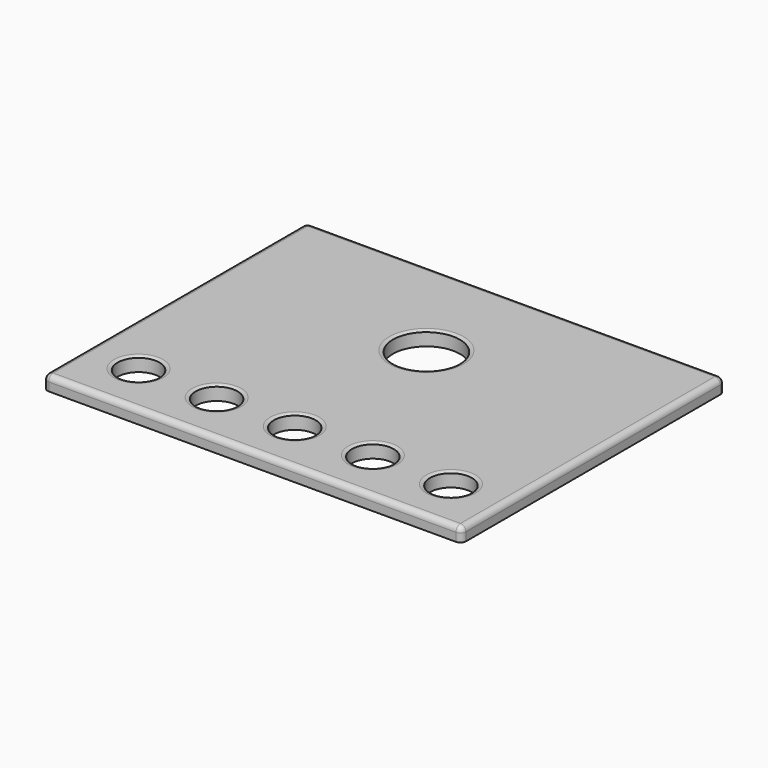
from build123d import *

# Parameters (mm, degrees)
F0_W         = 150
F0_H         = 118
F0_W_2       = 5
F0_H_2       = 5
F0_R         = 7.5
F0_R_2       = 12
F1_DEPTH     = 5
F2_DEPTH     = 1
F3_SIZE      = 0.5
F4_T1_DEPTH  = 160
F4_T3_DEPTH  = 128
F5_T1_DEPTH  = 8
F5_S5_W      = 2
F5_S5_H      = 2
F5_T6_DEPTH  = 2
F5_S11_W     = 2
F5_S11_H     = 2
F5_T12_DEPTH = 2
F5_S17_W     = 2
F5_S17_H     = 2
F5_T18_DEPTH = 2
F5_S23_W     = 2
F5_S23_H     = 2
F5_T24_DEPTH = 2


# Not quite as in the source:
# - a fillet or chamfer that OpenCascade refuses, or shapes differently, is made with other operations: its cross-section is extruded or revolved along the edge and cut away or added


with BuildPart() as f1:
    # F0 (on Top) → F1 (new body)
    with BuildSketch(Plane.XY):
        with Locations((0.2827864019, -6.098040469)):
            Rectangle(F0_W, F0_H)
        with Locations((-67.2172135981, -57.598040469)):
            Rectangle(F0_W_2, F0_H_2, mode=Mode.SUBTRACT)
        with Locations((-55.7172135981, -46.098040469)):
            Circle(F0_R, mode=Mode.SUBTRACT)
        with Locations((-27.7172135981, -46.098040469)):
            Circle(F0_R, mode=Mode.SUBTRACT)
        with Locations((0.2827864019, -46.098040469)):
            Circle(F0_R, mode=Mode.SUBTRACT)
        with Locations((28.2827864019, -46.098040469)):
            Circle(F0_R, mode=Mode.SUBTRACT)
        with Locations((67.7827864019, -57.598040469)):
            Rectangle(F0_W_2, F0_H_2, mode=Mode.SUBTRACT)
        with Locations((56.2827864019, -46.098040469)):
            Circle(F0_R, mode=Mode.SUBTRACT)
        with Locations((-67.2172135981, 45.401959531)):
            Rectangle(F0_W_2, F0_H_2, mode=Mode.SUBTRACT)
        with Locations((0.2827864019, 12.901959531)):
            Circle(F0_R_2, mode=Mode.SUBTRACT)
        with Locations((67.7827864019, 45.401959531)):
            Rectangle(F0_W_2, F0_H_2, mode=Mode.SUBTRACT)
        with Locations((-67.2172135981, -57.598040469)):
            Rectangle(F0_W_2, F0_H_2)
        with Locations((-67.2172135981, 45.401959531)):
            Rectangle(F0_W_2, F0_H_2)
        with Locations((67.7827864019, 45.401959531)):
            Rectangle(F0_W_2, F0_H_2)
        with Locations((67.7827864019, -57.598040469)):
            Rectangle(F0_W_2, F0_H_2)
    extrude(amount=F1_DEPTH)

    # F0 (on Top) → F2 (cut)
    with BuildSketch(Plane.XY):
        with Locations((-67.2172135981, 45.401959531)):
            Rectangle(F0_W_2, F0_H_2)
        with Locations((67.7827864019, 45.401959531)):
            Rectangle(F0_W_2, F0_H_2)
        with Locations((67.7827864019, -57.598040469)):
            Rectangle(F0_W_2, F0_H_2)
        with Locations((-67.2172135981, -57.598040469)):
            Rectangle(F0_W_2, F0_H_2)
    extrude(amount=F2_DEPTH, mode=Mode.SUBTRACT)

    # F3
    f3_edges = [f1.edges().sort_by_distance(p)[0] for p in [
        (-11.717214, 12.90196, 5),
        (-63.217214, -46.09804, 5),
        (-35.217214, -46.09804, 5),
        (-7.217214, -46.09804, 5),
        (20.782786, -46.09804, 5),
        (48.782786, -46.09804, 5),
    ]]
    chamfer(f3_edges, length=F3_SIZE)

    # F4: fillet of radius 2 on 10 edges, made by hand

    # F4_s2 → F4_t1 (cut)
    with BuildSketch(Plane.YZ.offset(-79.7172135981)):
        with BuildLine():
            ThreePointArc((50.901959531, 5), (52.3161730933, 4.4142135624), (52.901959531, 3))
            Line((52.901959531, 3), (52.901959531, 5))
            Line((52.901959531, 5), (50.901959531, 5))
        make_face()
        with BuildLine():
            ThreePointArc((-63.098040469, 5), (-64.5122540314, 4.4142135624), (-65.098040469, 3))
            Line((-65.098040469, 3), (-65.098040469, 5))
            Line((-65.098040469, 5), (-63.098040469, 5))
        make_face()
    extrude(amount=F4_T1_DEPTH, mode=Mode.SUBTRACT)

    # F4_s4 → F4_t3 (cut)
    with BuildSketch(Plane.XZ.offset(-57.901959531)):
        with BuildLine():
            ThreePointArc((-72.7172135981, 5), (-74.1314271605, 4.4142135624), (-74.7172135981, 3))
            Line((-74.7172135981, 3), (-74.7172135981, 5))
            Line((-74.7172135981, 5), (-72.7172135981, 5))
        make_face()
        with BuildLine():
            ThreePointArc((73.2827864019, 5), (74.6969999642, 4.4142135624), (75.2827864019, 3))
            Line((75.2827864019, 3), (75.2827864019, 5))
            Line((75.2827864019, 5), (73.2827864019, 5))
        make_face()
    extrude(amount=F4_T3_DEPTH, mode=Mode.SUBTRACT)

    # F4_s5 → F4_t6 (revolve, cut)
    with BuildSketch(Plane.XZ.offset(-12.901959531)):
        with BuildLine():
            ThreePointArc((13.6056620574, 5), (12.8985552762, 4.8708286934), (12.2827864019, 4.5))
            Line((12.2827864019, 4.5), (12.7827864019, 5))
            Line((12.7827864019, 5), (13.6056620574, 5))
        make_face()
    revolve(axis=Axis((0.2827864019, 12.901959531, 5), (0, 0, 1)), mode=Mode.SUBTRACT)

    # F4_s7 → F4_t8 (revolve, cut)
    with BuildSketch(Plane.XZ.offset(46.098040469)):
        with BuildLine():
            ThreePointArc((-46.8943379426, 5), (-47.6014447238, 4.8708286934), (-48.2172135981, 4.5))
            Line((-48.2172135981, 4.5), (-47.7172135981, 5))
            Line((-47.7172135981, 5), (-46.8943379426, 5))
        make_face()
    revolve(axis=Axis((-55.7172135981, -46.098040469, 5), (0, 0, 1)), mode=Mode.SUBTRACT)

    # F4_s9 → F4_t10 (revolve, cut)
    with BuildSketch(Plane.XZ.offset(46.098040469)):
        with BuildLine():
            ThreePointArc((-18.8943379426, 5), (-19.6014447238, 4.8708286934), (-20.2172135981, 4.5))
            Line((-20.2172135981, 4.5), (-19.7172135981, 5))
            Line((-19.7172135981, 5), (-18.8943379426, 5))
        make_face()
    revolve(axis=Axis((-27.7172135981, -46.098040469, 5), (0, 0, 1)), mode=Mode.SUBTRACT)

    # F4_s11 → F4_t12 (revolve, cut)
    with BuildSketch(Plane.XZ.offset(46.098040469)):
        with BuildLine():
            ThreePointArc((9.1056620574, 5), (8.3985552762, 4.8708286934), (7.7827864019, 4.5))
            Line((7.7827864019, 4.5), (8.2827864019, 5))
            Line((8.2827864019, 5), (9.1056620574, 5))
        make_face()
    revolve(axis=Axis((0.2827864019, -46.098040469, 5), (0, 0, 1)), mode=Mode.SUBTRACT)

    # F4_s13 → F4_t14 (revolve, cut)
    with BuildSketch(Plane.XZ.offset(46.098040469)):
        with BuildLine():
            ThreePointArc((37.1056620574, 5), (36.3985552762, 4.8708286934), (35.7827864019, 4.5))
            Line((35.7827864019, 4.5), (36.2827864019, 5))
            Line((36.2827864019, 5), (37.1056620574, 5))
        make_face()
    revolve(axis=Axis((28.2827864019, -46.098040469, 5), (0, 0, 1)), mode=Mode.SUBTRACT)

    # F4_s15 → F4_t16 (revolve, cut)
    with BuildSketch(Plane.XZ.offset(46.098040469)):
        with BuildLine():
            ThreePointArc((65.1056620574, 5), (64.3985552762, 4.8708286934), (63.7827864019, 4.5))
            Line((63.7827864019, 4.5), (64.2827864019, 5))
            Line((64.2827864019, 5), (65.1056620574, 5))
        make_face()
    revolve(axis=Axis((56.2827864019, -46.098040469, 5), (0, 0, 1)), mode=Mode.SUBTRACT)

    # F5: fillet of radius 2 on 14 edges, made by hand

    # F5_s2 → F5_t1 (cut)
    with BuildSketch(Plane.XY.offset(-5)):
        with BuildLine():
            ThreePointArc((73.2827864019, -65.098040469), (74.6969999642, -64.5122540314), (75.2827864019, -63.098040469))
            Line((75.2827864019, -63.098040469), (75.2827864019, -65.098040469))
            Line((75.2827864019, -65.098040469), (73.2827864019, -65.098040469))
        make_face()
        with BuildLine():
            ThreePointArc((-72.7172135981, -65.098040469), (-74.1314271605, -64.5122540314), (-74.7172135981, -63.098040469))
            Line((-74.7172135981, -63.098040469), (-74.7172135981, -65.098040469))
            Line((-74.7172135981, -65.098040469), (-72.7172135981, -65.098040469))
        make_face()
        with BuildLine():
            ThreePointArc((-74.7172135981, 50.901959531), (-74.1314271605, 52.3161730933), (-72.7172135981, 52.901959531))
            Line((-72.7172135981, 52.901959531), (-74.7172135981, 52.901959531))
            Line((-74.7172135981, 52.901959531), (-74.7172135981, 50.901959531))
        make_face()
        with BuildLine():
            ThreePointArc((75.2827864019, 50.901959531), (74.6969999642, 52.3161730933), (73.2827864019, 52.901959531))
            Line((73.2827864019, 52.901959531), (75.2827864019, 52.901959531))
            Line((75.2827864019, 52.901959531), (75.2827864019, 50.901959531))
        make_face()
    extrude(amount=F5_T1_DEPTH, mode=Mode.SUBTRACT)


with BuildPart() as f5_tool4:
    # F5_s5 → F5_t6 (new body)
    with BuildSketch(Plane.YZ.offset(73.2827864019)):
        with Locations((51.901959531, 4)):
            Rectangle(F5_S5_W, F5_S5_H)
    extrude(amount=F5_T6_DEPTH)

    # F5_s7 → F5_t8 (revolve, cut)
    with BuildSketch(Plane(origin=(73.2827864019, 50.901959531, 3), x_dir=(0, -0.7071067812, -0.7071067812), z_dir=(0, -0.7071067812, 0.7071067812))):
        with BuildLine():
            ThreePointArc((0, -2), (2, 0), (0, 2))
            Line((0, 2), (0, -2))
        make_face()
    revolve(axis=Axis((73.2827864019, 50.901959531, 3), (1, 0, 0)), mode=Mode.SUBTRACT)


with BuildPart() as f1_1:
    add(f1.part)

    # F5_t3: cut F5_tool4
    add(f5_tool4.part, mode=Mode.SUBTRACT)


with BuildPart() as f5_tool10:
    # F5_s11 → F5_t12 (new body)
    with BuildSketch(Plane.XZ.offset(63.098040469)):
        with Locations((74.2827864019, 4)):
            Rectangle(F5_S11_W, F5_S11_H)
    extrude(amount=F5_T12_DEPTH)

    # F5_s13 → F5_t14 (revolve, cut)
    with BuildSketch(Plane(origin=(73.2827864019, -63.098040469, 3), x_dir=(-0.7071067812, 0, -0.7071067812), z_dir=(-0.7071067812, 0, 0.7071067812))):
        with BuildLine():
            ThreePointArc((0, -2), (2, 0), (0, 2))
            Line((0, 2), (0, -2))
        make_face()
    revolve(axis=Axis((73.2827864019, -63.098040469, 3), (0, -1, 0)), mode=Mode.SUBTRACT)


with BuildPart() as f1_2:
    add(f1_1.part)

    # F5_t9: cut F5_tool10
    add(f5_tool10.part, mode=Mode.SUBTRACT)


with BuildPart() as f5_tool16:
    # F5_s17 → F5_t18 (new body)
    with BuildSketch(Plane.XZ.offset(63.098040469)):
        with Locations((-73.7172135981, 4)):
            Rectangle(F5_S17_W, F5_S17_H)
    extrude(amount=F5_T18_DEPTH)

    # F5_s19 → F5_t20 (revolve, cut)
    with BuildSketch(Plane(origin=(-72.7172135981, -63.098040469, 3), x_dir=(0.7071067812, 0, -0.7071067812), z_dir=(-0.7071067812, 0, -0.7071067812))):
        with BuildLine():
            ThreePointArc((0, -2), (2, 0), (0, 2))
            Line((0, 2), (0, -2))
        make_face()
    revolve(axis=Axis((-72.7172135981, -63.098040469, 3), (0, -1, 0)), mode=Mode.SUBTRACT)


with BuildPart() as f1_3:
    add(f1_2.part)

    # F5_t15: cut F5_tool16
    add(f5_tool16.part, mode=Mode.SUBTRACT)


with BuildPart() as f5_tool22:
    # F5_s23 → F5_t24 (new body)
    with BuildSketch(Plane.YZ.offset(-72.7172135981)):
        with Locations((51.901959531, 4)):
            Rectangle(F5_S23_W, F5_S23_H)
    extrude(amount=-F5_T24_DEPTH)

    # F5_s25 → F5_t26 (revolve, cut)
    with BuildSketch(Plane(origin=(-72.7172135981, 50.901959531, 3), x_dir=(0, -0.7071067812, -0.7071067812), z_dir=(0, 0.7071067812, -0.7071067812))):
        with BuildLine():
            ThreePointArc((0, -2), (2, 0), (0, 2))
            Line((0, 2), (0, -2))
        make_face()
    revolve(axis=Axis((-72.7172135981, 50.901959531, 3), (-1, 0, 0)), mode=Mode.SUBTRACT)


with BuildPart() as f1_4:
    add(f1_3.part)

    # F5_t21: cut F5_tool22
    add(f5_tool22.part, mode=Mode.SUBTRACT)


solid = f1_4.part
